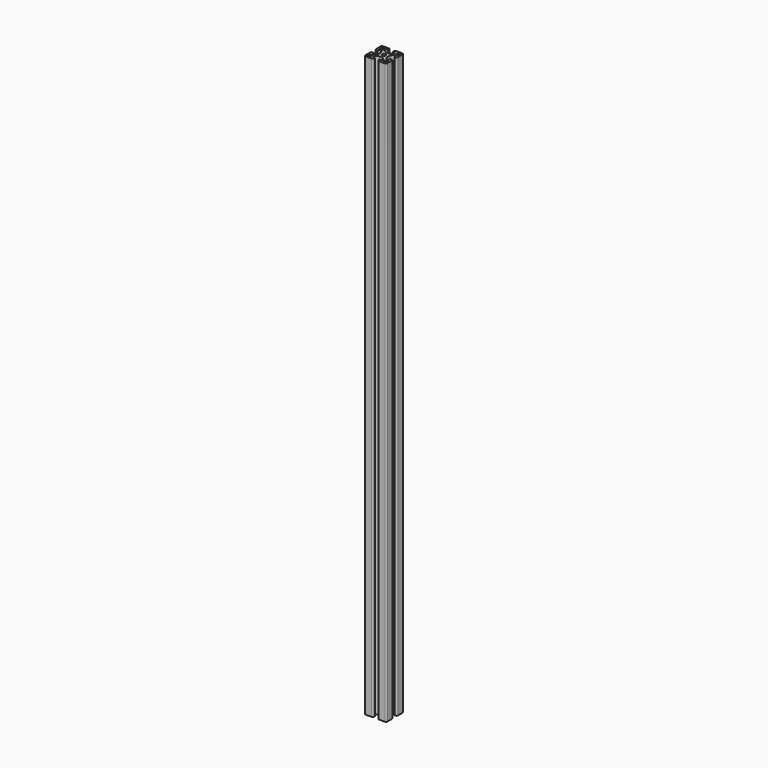
from build123d import *

# Parameters (mm, degrees)
F0_R     = 3.4
F1_DEPTH = 1060


# Not quite as in the source:
# - ends of sketch curves that miss each other by under 0.0002 mm in the source are joined


with BuildPart() as f1:
    # F0 (on Top) → F1 (new body)
    with BuildSketch(Plane.XY):
        with BuildLine():
            ThreePointArc((-37.8290628647, 13.3437199509), (-39.194573333, 10.8017277117), (-41.229063, 8.755464))
            ThreePointArc((-41.229063, 8.755464), (-43.8470969887, 8.5193960225), (-45.229063, 10.755464))
            Line((-45.229063, 10.755464), (-45.229063, 12.055464))
            ThreePointArc((-45.229063, 12.055464), (-45.3755096094, 12.4090173906), (-45.729063, 12.555464))
            Line((-45.729063, 12.555464), (-47.229063, 12.555464))
            ThreePointArc((-47.229063, 12.555464), (-48.996829953, 11.823230953), (-49.729063, 10.055464))
            Line((-49.729063, 10.055464), (-49.729063, -0.744536))
            ThreePointArc((-49.729063, -0.744536), (-48.996829953, -2.512302953), (-47.229063, -3.244536))
            Line((-47.229063, -3.244536), (-36.429063, -3.244536))
            ThreePointArc((-36.429063, -3.244536), (-34.661296047, -2.512302953), (-33.929063, -0.744536))
            Line((-33.929063, -0.744536), (-33.929063, 0.755464))
            ThreePointArc((-33.929063, 0.755464), (-34.0755096094, 1.1090173906), (-34.429063, 1.255464))
            Line((-34.429063, 1.255464), (-35.729063, 1.255464))
            ThreePointArc((-35.729063, 1.255464), (-37.9651309775, 2.6374300113), (-37.729063, 5.255464))
            ThreePointArc((-37.729063, 5.255464), (-35.6827992883, 7.289953667), (-33.1408070491, 8.6554641353))
            ThreePointArc((-33.1408070491, 8.6554641353), (-32.7208836531, 8.767678459), (-32.287871, 8.805464))
            Line((-32.287871, 8.805464), (-27.170255, 8.805464))
            ThreePointArc((-27.170255, 8.805464), (-26.7372423469, 8.767678459), (-26.3173189877, 8.6554640338))
            ThreePointArc((-26.3173189877, 8.6554640338), (-23.7753267117, 7.289953667), (-21.729063, 5.255464))
            ThreePointArc((-21.729063, 5.255464), (-21.4929950225, 2.6374300113), (-23.729063, 1.255464))
            Line((-23.729063, 1.255464), (-25.029063, 1.255464))
            ThreePointArc((-25.029063, 1.255464), (-25.3826163906, 1.1090173906), (-25.529063, 0.755464))
            Line((-25.529063, 0.755464), (-25.529063, -0.744536))
            ThreePointArc((-25.529063, -0.744536), (-24.796829953, -2.512302953), (-23.029063, -3.244536))
            Line((-23.029063, -3.244536), (-12.229063, -3.244536))
            ThreePointArc((-12.229063, -3.244536), (-10.461296047, -2.512302953), (-9.729063, -0.744536))
            Line((-9.729063, -0.744536), (-9.729063, 10.055464))
            ThreePointArc((-9.729063, 10.055464), (-10.461296047, 11.823230953), (-12.229063, 12.555464))
            Line((-12.229063, 12.555464), (-13.729063, 12.555464))
            ThreePointArc((-13.729063, 12.555464), (-14.0826163906, 12.4090173906), (-14.229063, 12.055464))
            Line((-14.229063, 12.055464), (-14.229063, 10.755464))
            ThreePointArc((-14.229063, 10.755464), (-15.6110290113, 8.5193960225), (-18.229063, 8.755464))
            ThreePointArc((-18.229063, 8.755464), (-20.263552667, 10.8017277117), (-21.6290631353, 13.3437199509))
            ThreePointArc((-21.6290631353, 13.3437199509), (-21.741277459, 13.7636433469), (-21.779063, 14.196656))
            Line((-21.779063, 14.196656), (-21.779063, 19.314273))
            ThreePointArc((-21.779063, 19.314273), (-21.741277459, 19.7472856531), (-21.6290630338, 20.1672090123))
            ThreePointArc((-21.6290630338, 20.1672090123), (-20.2635523872, 22.7092006659), (-18.229063, 24.755464))
            ThreePointArc((-18.229063, 24.755464), (-15.6110290113, 24.9915319775), (-14.229063, 22.755464))
            Line((-14.229063, 22.755464), (-14.229063, 21.455464))
            ThreePointArc((-14.229063, 21.455464), (-14.0826163906, 21.1019106094), (-13.729063, 20.955464))
            Line((-13.729063, 20.955464), (-12.229063, 20.955464))
            ThreePointArc((-12.229063, 20.955464), (-10.461296047, 21.687697047), (-9.729063, 23.455464))
            Line((-9.729063, 23.455464), (-9.729063, 34.255464))
            ThreePointArc((-9.729063, 34.255464), (-10.461296047, 36.023230953), (-12.229063, 36.755464))
            Line((-12.229063, 36.755464), (-23.029063, 36.755464))
            ThreePointArc((-23.029063, 36.755464), (-24.796829953, 36.023230953), (-25.529063, 34.255464))
            Line((-25.529063, 34.255464), (-25.529063, 32.755464))
            ThreePointArc((-25.529063, 32.755464), (-25.3826163906, 32.4019106094), (-25.029063, 32.255464))
            Line((-25.029063, 32.255464), (-23.729063, 32.255464))
            ThreePointArc((-23.729063, 32.255464), (-21.4929950225, 30.8734979887), (-21.729063, 28.255464))
            ThreePointArc((-21.729063, 28.255464), (-23.7753267117, 26.220974333), (-26.3173189509, 24.8554638647))
            ThreePointArc((-26.3173189509, 24.8554638647), (-26.7372423469, 24.743249541), (-27.170255, 24.705464))
            Line((-27.170255, 24.705464), (-32.287871, 24.705464))
            ThreePointArc((-32.287871, 24.705464), (-32.7208836531, 24.743249541), (-33.1408070123, 24.8554639662))
            ThreePointArc((-33.1408070123, 24.8554639662), (-35.6827992883, 26.220974333), (-37.729063, 28.255464))
            ThreePointArc((-37.729063, 28.255464), (-37.9651309775, 30.8734979887), (-35.729063, 32.255464))
            Line((-35.729063, 32.255464), (-34.429063, 32.255464))
            ThreePointArc((-34.429063, 32.255464), (-34.0755096094, 32.4019106094), (-33.929063, 32.755464))
            Line((-33.929063, 32.755464), (-33.929063, 34.255464))
            ThreePointArc((-33.929063, 34.255464), (-34.661296047, 36.023230953), (-36.429063, 36.755464))
            Line((-36.429063, 36.755464), (-47.229063, 36.755464))
            ThreePointArc((-47.229063, 36.755464), (-48.996829953, 36.023230953), (-49.729063, 34.255464))
            Line((-49.729063, 34.255464), (-49.729063, 23.455464))
            ThreePointArc((-49.729063, 23.455464), (-48.996829953, 21.687697047), (-47.229063, 20.955464))
            Line((-47.229063, 20.955464), (-45.729063, 20.955464))
            ThreePointArc((-45.729063, 20.955464), (-45.3755096094, 21.1019106094), (-45.229063, 21.455464))
            Line((-45.229063, 21.455464), (-45.229063, 22.755464))
            ThreePointArc((-45.229063, 22.755464), (-43.8470969887, 24.9915319775), (-41.229063, 24.755464))
            ThreePointArc((-41.229063, 24.755464), (-39.1945736128, 22.7092006659), (-37.8290631854, 20.1672089327))
            ThreePointArc((-37.8290631854, 20.1672089327), (-37.716848541, 19.7472856531), (-37.679063, 19.314273))
            Line((-37.679063, 19.314273), (-37.679063, 14.196656))
            ThreePointArc((-37.679063, 14.196656), (-37.716848541, 13.7636433469), (-37.8290628647, 13.3437199509))
        make_face()
        Polygon((-43.257983, -0.764408), (-45.929556, -0.764408), (-46.636663, -1.471515), (-48.050877, -0.057301), (-47.34377, 0.649805), (-47.34377, 3.321378), (-48.050877, 4.028485), (-46.636663, 5.442699), (-45.929556, 4.735592), (-43.257983, 4.735592), (-42.550877, 5.442699), (-41.136663, 4.028485), (-41.84377, 3.321378), (-41.84377, 0.649805), (-41.136663, -0.057301), (-42.550877, -1.471515), align=None, mode=Mode.SUBTRACT)
        Polygon((-12.20919, 3.226544), (-12.20919, 0.554971), (-11.502084, -0.152136), (-12.916297, -1.566349), (-13.623404, -0.859242), (-16.294977, -0.859242), (-17.002084, -1.566349), (-18.416297, -0.152136), (-17.70919, 0.554971), (-17.70919, 3.226544), (-18.416297, 3.933651), (-17.002084, 5.347864), (-16.294977, 4.640758), (-13.623404, 4.640758), (-12.916297, 5.347864), (-11.502084, 3.933651), align=None, mode=Mode.SUBTRACT)
        with Locations((-29.729063, 16.755464)):
            Circle(F0_R, mode=Mode.SUBTRACT)
        Polygon((-47.248935, 30.284385), (-47.248935, 32.955957), (-47.956042, 33.663064), (-46.541829, 35.077278), (-45.834722, 34.370171), (-43.163149, 34.370171), (-42.456042, 35.077278), (-41.041829, 33.663064), (-41.748935, 32.955957), (-41.748935, 30.284385), (-41.041829, 29.577278), (-42.456042, 28.163064), (-43.163149, 28.870171), (-45.834722, 28.870171), (-46.541829, 28.163064), (-47.956042, 29.577278), align=None, mode=Mode.SUBTRACT)
        Polygon((-16.200143, 34.275337), (-13.52857, 34.275337), (-12.821463, 34.982444), (-11.407249, 33.56823), (-12.114356, 32.861123), (-12.114356, 30.18955), (-11.407249, 29.482444), (-12.821463, 28.06823), (-13.52857, 28.775337), (-16.200143, 28.775337), (-16.907249, 28.06823), (-18.321463, 29.482444), (-17.614356, 30.18955), (-17.614356, 32.861123), (-18.321463, 33.56823), (-16.907249, 34.982444), align=None, mode=Mode.SUBTRACT)
    extrude(amount=F1_DEPTH)


solid = f1.part
